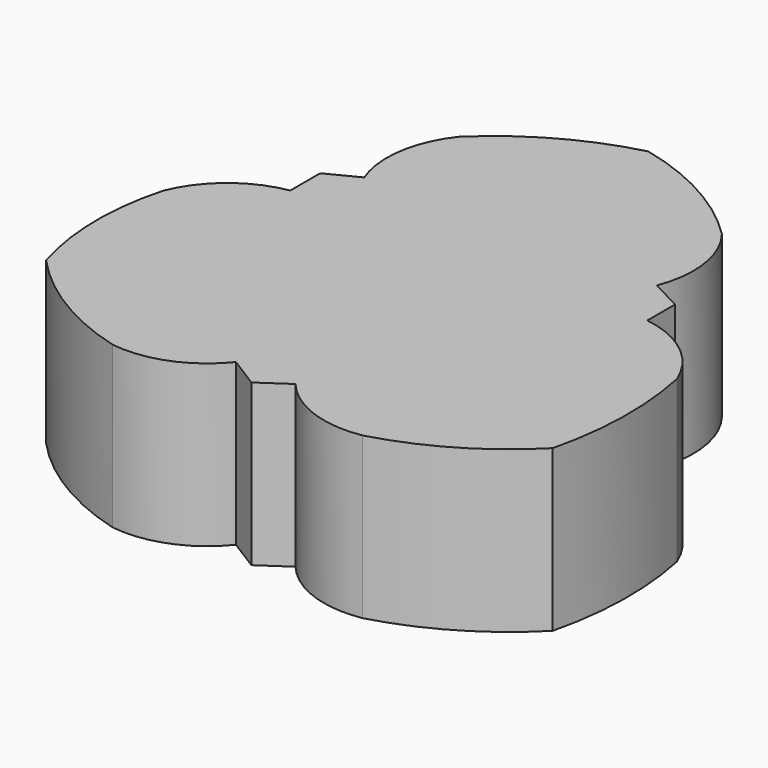
from build123d import *

# Parameters (mm, degrees)
F1_DEPTH = 11.1125


# Not quite as in the source:
# - a length typed as a fraction of an inch, garbled in the dataset ("3 / 203.2 mm" for 3/8 in), is restored


with BuildPart() as f1:
    # F0 (on Top) → F1 (new body)
    with BuildSketch(Plane.XY):
        with BuildLine():
            ThreePointArc((-0.1411418198, 20.1985444874), (-5.0054503986, 18.2564119782), (-9.2097157612, 15.1327075437))
            ThreePointArc((-9.2097157612, 15.1327075437), (-10.6205392688, 11.8246856933), (-10.2093555033, 8.2519613206))
            Line((-10.2093555033, 8.2519613206), (-12.369341217, 7.1464567445))
            Line((-12.369341217, 7.1464567445), (-12.369341217, 4.6386048198))
            Line((-12.369341217, 4.6386048198), (-12.369341217, 4.5682978211))
            ThreePointArc((-12.369341217, 4.5682978211), (-15.5930977879, 3.1185654947), (-17.7027139134, 0.2823972963))
            ThreePointArc((-17.7027139134, 0.2823972963), (-18.3641606661, -4.889059653), (-17.5542831421, -10.0393583998))
            ThreePointArc((-17.5542831421, -10.0393583998), (-13.4613837791, -13.3941238354), (-8.5996589687, -15.484556372))
            ThreePointArc((-8.5996589687, -15.484556372), (-5.0294162563, -15.0523544446), (-2.1409380715, -12.9098966718))
            Line((-2.1409380715, -12.9098966718), (0, -14.2561570176))
            Line((0, -14.2561570176), (1.9696742658, -12.9098966718))
            ThreePointArc((1.9696742658, -12.9098966718), (4.9392756736, -15.0084468105), (8.560301624, -15.3410370587))
            ThreePointArc((8.560301624, -15.3410370587), (13.367982191, -13.3015402533), (17.4874793738, -10.0916987285))
            ThreePointArc((17.4874793738, -10.0916987285), (18.16772005, -4.8427956267), (17.6633565687, 0.4259166096))
            ThreePointArc((17.6633565687, 0.4259166096), (15.4847616458, 3.3168082822), (12.1560195839, 4.739132713))
            Line((12.1560195839, 4.739132713), (12.1560195839, 7.1464567445))
            Line((12.1560195839, 7.1464567445), (9.9960338703, 8.2519613206))
            ThreePointArc((9.9960338703, 8.2519613206), (10.4072176357, 11.8246856933), (8.9963941282, 15.1327075437))
            ThreePointArc((8.9963941282, 15.1327075437), (4.7823081966, 18.3053860292), (-0.1411418198, 20.1985444874))
        make_face()
    extrude(amount=F1_DEPTH)


solid = f1.part
